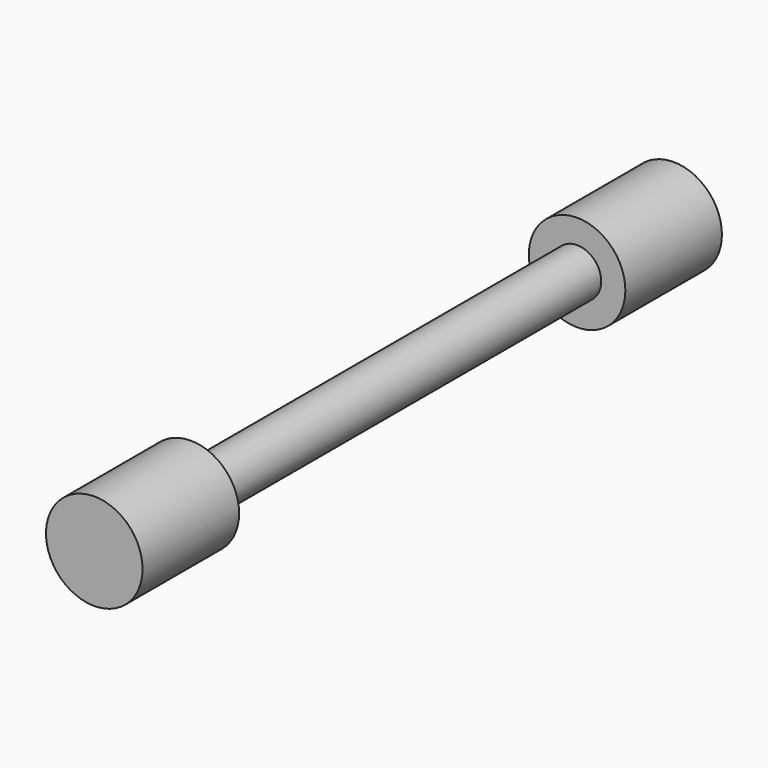
from build123d import *

# Parameters (mm, degrees)
F0_R          = 5
F1_DEPTH      = 50
F1_DEPTH_BACK = 50
F2_R          = 10
F3_DEPTH      = 25


# Not quite as in the source:
# - a pattern or mirror of a feature is missing from the dataset's text; its kind, count and spacing are read off the source's solid


with BuildPart() as f1:
    # F0 (on Front) → F1 (new body, two sides)
    with BuildSketch(Plane.XZ) as f1_sk:
        Circle(F0_R)
    extrude(amount=F1_DEPTH)
    extrude(f1_sk.sketch, amount=-F1_DEPTH_BACK)

    # F2 (on face) → F3 (join)
    with BuildSketch(Plane.XZ.offset(50)):
        Circle(F2_R)
    f3 = extrude(amount=F3_DEPTH)

    # F3_copies: F3 across plane
    add(f3.mirror(Plane.ZX))


solid = f1.part
